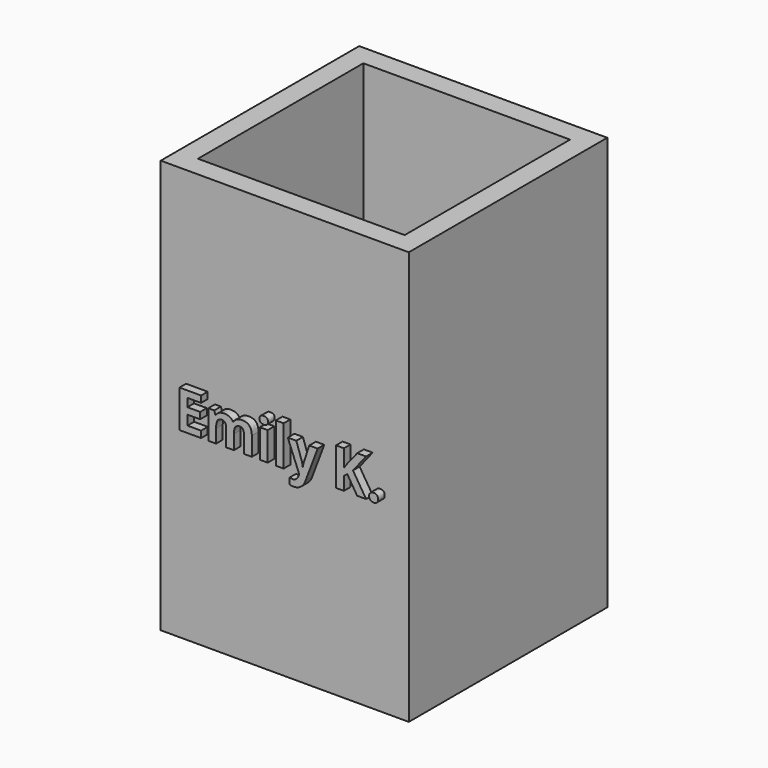
from build123d import *

# Parameters (mm, degrees)
F0_W         = 76.2
F0_H         = 127
F1_DEPTH     = 76.2
F2_W         = 63.5
F2_H         = 63.5
F3_DEPTH     = 120.65
F4_TEXT_SIZE = 16.1257043092
F5_DEPTH     = 2.54


# Not quite as in the source:
# - Text() gives the source's letters only with a copy of the font that has no kerning and outlines rounded to 1/6400 em; it was checked with that copy


with BuildPart() as f1:
    # F0 (on Front) → F1 (new body)
    with BuildSketch(Plane.XZ):
        with Locations((-5.6387065772, 38.4621014678)):
            Rectangle(F0_W, F0_H)
    extrude(amount=F1_DEPTH)

    # F2 (on face) → F3 (cut)
    with BuildSketch(Plane.XY.offset(101.9621014678)):
        with Locations((-5.6387065772, -38.1)):
            Rectangle(F2_W, F2_H)
    extrude(amount=-F3_DEPTH, mode=Mode.SUBTRACT)

    # F4 (on face) → F5 (join)
    with BuildSketch(Plane.XZ.offset(76.2)):
        with Locations((-37.3887065772, 32.6582014678)):
            Text('Emily K.', F4_TEXT_SIZE, font='Open Sans', font_style=FontStyle.BOLD, text_align=(TextAlign.LEFT, TextAlign.BOTTOM))
    extrude(amount=F5_DEPTH)


solid = f1.part
